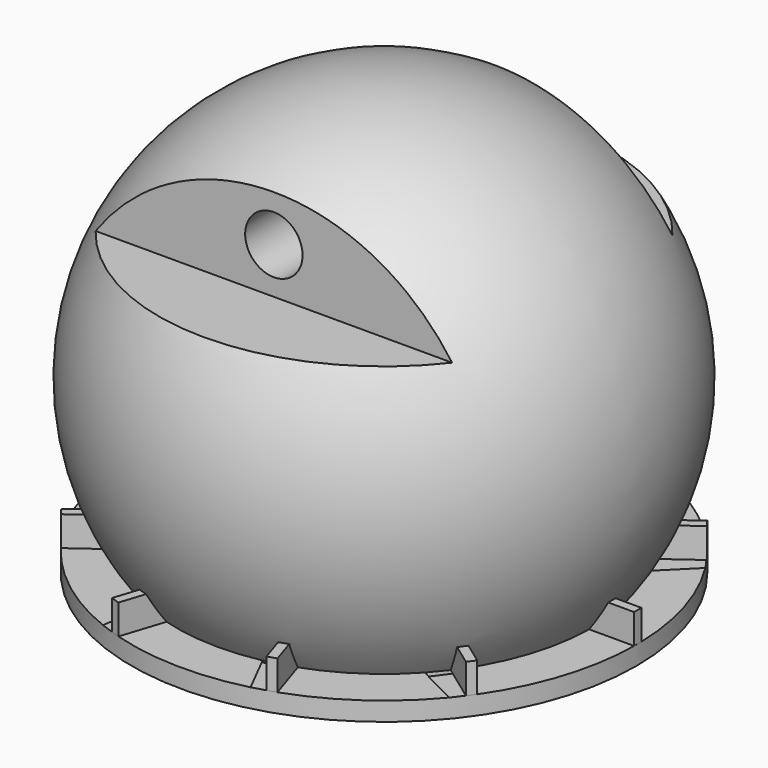
from build123d import *

# Parameters (mm, degrees)
F3_DEPTH        = 1.651
F3_COPIES_COUNT = 10
F6_W            = 25.4
F6_H            = 5.08
F7_DEPTH        = 6.35
F8_R            = 1.5875
F9_DEPTH        = 3.81
F9_DEPTH_BACK   = 19.05
F10_R           = 9.906
F11_DEPTH       = 12.7
F12_R           = 9.525
F13_DEPTH       = 57.15
F14_R           = 7.62
F15_DEPTH       = 44.45


# Not quite as in the source:
# - a feature of the source that left no trace in its solid (it failed there, or was rolled back) is left out
# - a pattern or mirror of a feature is missing from the dataset's text; its kind, count and spacing are read off the source's solid


with BuildPart() as f1:
    # F0 (on Front) → F1 (revolve)
    with BuildSketch(Plane.XZ):
        with BuildLine():
            Line((-43.18, 1.016), (-45.6726494673, 1.016))
            ThreePointArc((-45.6726494673, 1.016), (-44.3886326409, 15.9499637645), (-57.15, 23.8125))
            Line((-57.15, 23.8125), (-57.15, -0.0228488987))
            Line((-57.15, -0.0228488987), (-43.18, -0.0228488987))
            Line((-43.18, -0.0228488987), (-43.18, 1.016))
        make_face()
    revolve(axis=Axis((-57.15, 0, 11.8948255506), (0, 0, 1)))

    # F2 (on face) → F3 (join)
    with BuildSketch(Plane.XY.offset(1.016)):
        with BuildLine():
            ThreePointArc((-45.6726494673, 0), (-45.6729398633, -0.081644771), (-45.6738110366, -0.1632854104))
            Line((-45.6738110366, -0.1632854104), (-43.1842536235, -0.1632854104))
            Line((-43.1842536235, -0.1632854104), (-43.1842536235, 0.3447145896))
            Line((-43.1842536235, 0.3447145896), (-45.6738110366, 0.3447145896))
            Line((-45.6738110366, 0.3447145896), (-45.6738110366, 0.1632854104))
            ThreePointArc((-45.6738110366, 0.1632854104), (-45.6729398633, 0.081644771), (-45.6726494673, 0))
        make_face()
    f3 = extrude(amount=F3_DEPTH)

    # F3_copies: F3 ×10 about axis
    f3_copies_axis = Axis((-57.15, 0, 0), (0, 0, 1))
    for i in range(1, F3_COPIES_COUNT):
        add(f3.rotate(f3_copies_axis, i * 360 / F3_COPIES_COUNT))

    # F6 (on offset) → F7 (cut)
    with BuildSketch(Plane.XY.offset(16.51)):
        with Locations((-57.15, 10.16)):
            Rectangle(F6_W, F6_H)
        with Locations((-57.15, -10.16)):
            Rectangle(F6_W, F6_H)
    extrude(amount=F7_DEPTH, mode=Mode.SUBTRACT)

    # F8 (on face) → F9 (cut, two sides)
    with BuildSketch(Plane.XZ.offset(7.62)) as f9_sk:
        with Locations((-57.15, 19.05)):
            Circle(F8_R)
    extrude(amount=F9_DEPTH, mode=Mode.SUBTRACT)
    extrude(f9_sk.sketch, amount=-F9_DEPTH_BACK, mode=Mode.SUBTRACT)

    # F10 (on face) → F11 (cut)
    with BuildSketch(Plane(origin=(0, 0, -0.0228488987), x_dir=(1, 0, 0), z_dir=(0, 0, -1))):
        with Locations((-57.15, 0)):
            Circle(F10_R)
    extrude(amount=-F11_DEPTH, mode=Mode.SUBTRACT)


with BuildPart() as f13:
    # F12 (on Top) → F13 (new body)
    with BuildSketch(Plane.XY):
        Circle(F12_R)
    extrude(amount=F13_DEPTH)

    # F14 (on face) → F15 (cut)
    with BuildSketch(Plane(origin=(0, 0, 0), x_dir=(1, 0, 0), z_dir=(0, 0, -1))):
        Circle(F14_R)
    extrude(amount=-F15_DEPTH, mode=Mode.SUBTRACT)


solid = f1.part
